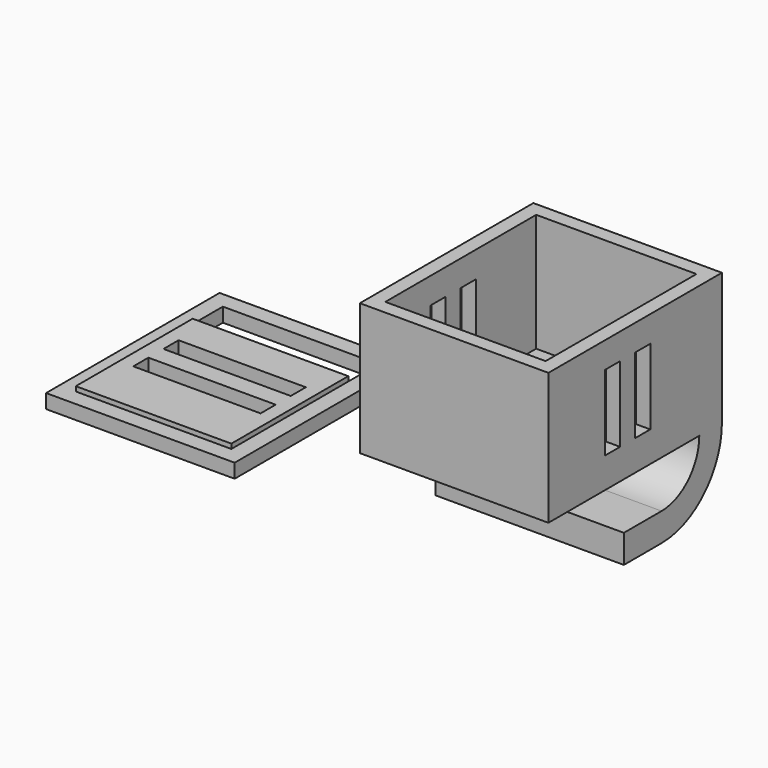
from build123d import *

# Parameters (mm, degrees)
F0_W     = 20
F0_H     = 23
F0_W_2   = 17
F0_H_2   = 20
F1_DEPTH = 14
F2_DEPTH = 1.5
F3_W     = 20
F3_H     = 23
F4_DEPTH = 1.5
F3_W_2   = 16.5
F3_H_2   = 15.5
F3_W_3   = 13.5
F3_H_3   = 2
F5_DEPTH = 2
F6_W     = 2
F6_H     = 8
F6_H_2   = 8.00022727
F7_DEPTH = 25
F8_W     = 5
F8_H     = 3
F9_DEPTH = 20


# Not quite as in the source:
# - a feature names something its author has since deleted; it is built from what else it names


with BuildPart() as f1:
    # F0 (on Top) → F1 (new body)
    with BuildSketch(Plane.XY):
        with Locations((-0.2807364799, -3.5512268197)):
            Rectangle(F0_W, F0_H)
        with Locations((-0.2807364799, -3.5512268197)):
            Rectangle(F0_W_2, F0_H_2, mode=Mode.SUBTRACT)
    extrude(amount=F1_DEPTH)

    # F0 (on Top) → F2 (join)
    with BuildSketch(Plane.XY):
        with Locations((-0.2807364799, -3.5512268197)):
            Rectangle(F0_W_2, F0_H_2)
    extrude(amount=F2_DEPTH)

    # F6 (on face) → F7 (cut)
    with BuildSketch(Plane(origin=(-10.2807364799, 0, 0), x_dir=(0, -1, 0), z_dir=(-1, 0, 0))):
        with Locations((2.5512268197, 7.2315260049)):
            Rectangle(F6_W, F6_H)
        with Locations((6.5512268197, 7.2316396399)):
            Rectangle(F6_W, F6_H_2)
    extrude(amount=-F7_DEPTH, mode=Mode.SUBTRACT)

    # F8 (on face) → F9 (join)
    with BuildSketch(Plane(origin=(-10.2807364799, 0, 0), x_dir=(0, -1, 0), z_dir=(-1, 0, 0))):
        with BuildLine():
            ThreePointArc((0.0512268197, -5), (-3.4843070863, -3.5355339059), (-4.9487731803, 0))
            Line((-4.9487731803, 0), (-7.9487731803, 0))
            ThreePointArc((-7.9487731803, 0), (-5.6056274298, -5.6568542495), (0.0512268197, -8))
            Line((0.0512268197, -8), (0.0512268197, -5))
        make_face()
        with Locations((2.5512268197, -6.5)):
            Rectangle(F8_W, F8_H)
    extrude(amount=-F9_DEPTH)


with BuildPart() as f4:
    # F3 (on Top) → F4 (new body)
    with BuildSketch(Plane.XY):
        with Locations((-25.5064666271, -13.6185353845)):
            Rectangle(F3_W, F3_H)
        Polygon((-33.7564666271, -7.8685353845), (-33.7564666271, -3.8685353845), (-17.2564666271, -3.8685353845), (-17.2564666271, -7.8685353845), (-17.2564666271, -23.3685353845), (-33.7564666271, -23.3685353845), align=None, mode=Mode.SUBTRACT)
    extrude(amount=F4_DEPTH)

    # F3 (on Top) → F5 (join)
    with BuildSketch(Plane.XY):
        with Locations((-25.5064666271, -15.6185353845)):
            Rectangle(F3_W_2, F3_H_2)
        with Locations((-25.5064666271, -16.6185353845)):
            Rectangle(F3_W_3, F3_H_3, mode=Mode.SUBTRACT)
        with Locations((-25.5064666271, -12.6185353845)):
            Rectangle(F3_W_3, F3_H_3, mode=Mode.SUBTRACT)
    extrude(amount=F5_DEPTH)


solid = Compound([f1.part, f4.part])
